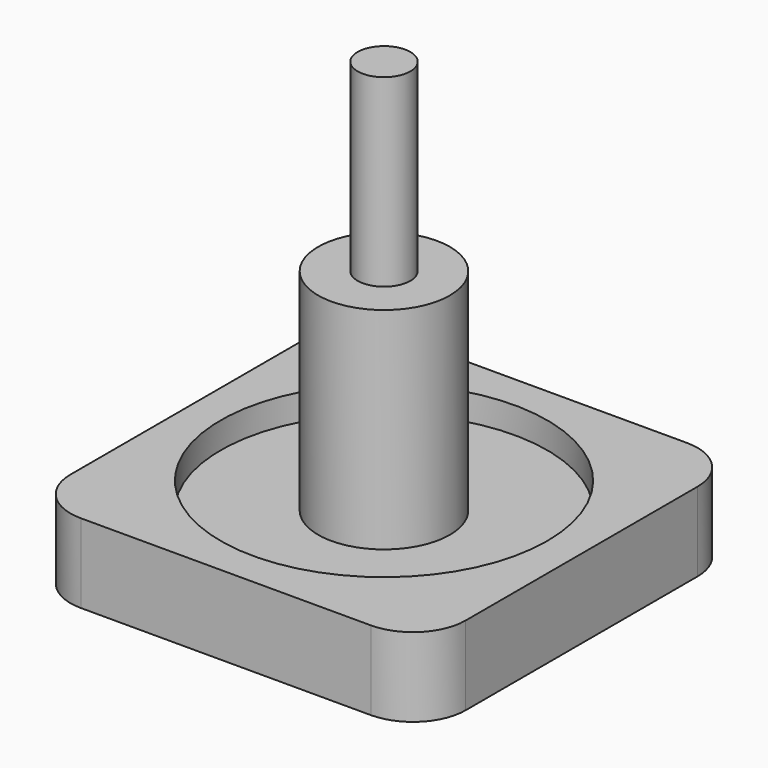
from build123d import *

# Parameters (mm, degrees)
F0_R     = 2.5
F1_DEPTH = 8
F2_R     = 1
F3_DEPTH = 7
F4_R     = 2.5
F5_DEPTH = 2
F6_R     = 6.2
F7_DEPTH = 1


with BuildPart() as f1:
    # F0 (on Top) → F1 (new body)
    with BuildSketch(Plane.XY):
        Circle(F0_R)
    extrude(amount=F1_DEPTH)

    # F2 (on face) → F3 (join)
    with BuildSketch(Plane.XY.offset(8)):
        Circle(F2_R)
    extrude(amount=F3_DEPTH)

    # F4 (on face) → F5 (join)
    with BuildSketch(Plane(origin=(0, 0, 0), x_dir=(1, 0, 0), z_dir=(0, 0, -1))):
        with BuildLine():
            Line((5.5, 7.5), (-5.5, 7.5))
            ThreePointArc((-5.5, 7.5), (-6.9142135624, 6.9142135624), (-7.5, 5.5))
            Line((-7.5, 5.5), (-7.5, -5.5))
            ThreePointArc((-7.5, -5.5), (-6.9142135624, -6.9142135624), (-5.5, -7.5))
            Line((-5.5, -7.5), (5.5, -7.5))
            ThreePointArc((5.5, -7.5), (6.9142135624, -6.9142135624), (7.5, -5.5))
            Line((7.5, -5.5), (7.5, 5.5))
            ThreePointArc((7.5, 5.5), (6.9142135624, 6.9142135624), (5.5, 7.5))
        make_face()
        Circle(F4_R, mode=Mode.SUBTRACT)
        Circle(F4_R)
    extrude(amount=F5_DEPTH)

    # F6 (on face) → F7 (join)
    with BuildSketch(Plane.XY):
        with BuildLine():
            Line((5.5, 7.5), (-5.5, 7.5))
            ThreePointArc((-5.5, 7.5), (-6.9142135624, 6.9142135624), (-7.5, 5.5))
            Line((-7.5, 5.5), (-7.5, -5.5))
            ThreePointArc((-7.5, -5.5), (-6.9142135624, -6.9142135624), (-5.5, -7.5))
            Line((-5.5, -7.5), (5.5, -7.5))
            ThreePointArc((5.5, -7.5), (6.9142135624, -6.9142135624), (7.5, -5.5))
            Line((7.5, -5.5), (7.5, 5.5))
            ThreePointArc((7.5, 5.5), (6.9142135624, 6.9142135624), (5.5, 7.5))
        make_face()
        Circle(F6_R, mode=Mode.SUBTRACT)
    extrude(amount=F7_DEPTH)


solid = f1.part
